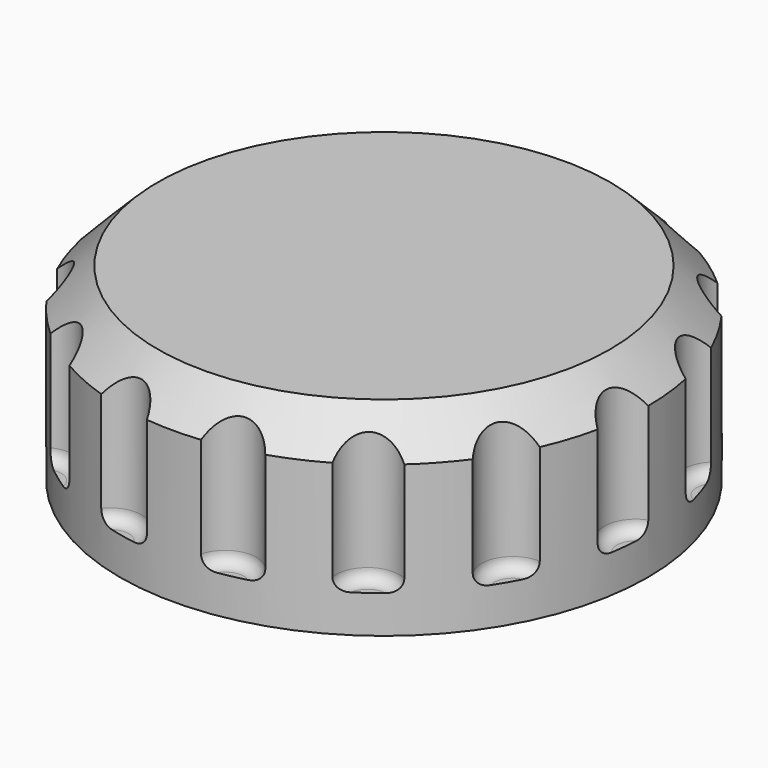
from build123d import *

# Parameters (mm, degrees)
F0_R         = 21
F1_DEPTH     = 15
F2_R         = 2.5
F3_DEPTH     = 12
F4_T3_ANGLE  = 241.487040257
F4_S4_R      = 21
F4_T5_DEPTH  = 5
F4_T8_ANGLE  = 241.487040257
F4_S9_R      = 21
F4_T10_DEPTH = 5
F4_T13_ANGLE = 241.487040257
F4_S14_R     = 21
F4_T15_DEPTH = 5
F4_T18_ANGLE = 241.487040257
F4_S19_R     = 21
F4_T20_DEPTH = 5
F4_T23_ANGLE = 241.487040257
F4_S24_R     = 21
F4_T25_DEPTH = 5
F4_T28_ANGLE = 241.487040257
F4_S29_R     = 21
F4_T30_DEPTH = 5
F4_T33_ANGLE = 241.487040257
F4_S34_R     = 21
F4_T35_DEPTH = 5
F4_T38_ANGLE = 241.487040257
F4_S39_R     = 21
F4_T40_DEPTH = 5
F4_T43_ANGLE = 241.487040257
F4_S44_R     = 21
F4_T45_DEPTH = 5
F4_T48_ANGLE = 241.487040257
F4_S49_R     = 21
F4_T50_DEPTH = 5
F4_T53_ANGLE = 241.487040257
F4_S54_R     = 21
F4_T55_DEPTH = 5
F4_T58_ANGLE = 241.487040257
F4_S59_R     = 21
F4_T60_DEPTH = 5
F4_T63_ANGLE = 241.487040257
F4_S64_R     = 21
F4_T65_DEPTH = 5
F4_T68_ANGLE = 241.487040257
F4_S69_R     = 21
F4_T70_DEPTH = 5
F4_T73_ANGLE = 241.487040257
F4_S74_R     = 21
F4_T75_DEPTH = 5
F5_T2_ANGLE  = 53.8780203583
F5_T4_ANGLE  = 53.8780203583
F5_T6_ANGLE  = 53.8780203583
F5_T8_ANGLE  = 53.8780203583
F5_T10_ANGLE = 53.8780203583
F5_T12_ANGLE = 53.8780203583
F5_T14_ANGLE = 53.8780203583
F5_T16_ANGLE = 53.8780203583
F5_T18_ANGLE = 53.8780203583
F5_T20_ANGLE = 53.8780203583
F5_T22_ANGLE = 53.8780203583
F5_T24_ANGLE = 53.8780203583
F5_T26_ANGLE = 53.8780203583
F5_T28_ANGLE = 53.8780203583
F5_T30_ANGLE = 53.8780203583


# Not quite as in the source:
# - a fillet or chamfer that OpenCascade refuses, or shapes differently, is made with other operations: its cross-section is extruded or revolved along the edge and cut away or added


with BuildPart() as f1:
    # F0 (on Top) → F1 (new body)
    with BuildSketch(Plane.XY):
        Circle(F0_R)
    extrude(amount=F1_DEPTH)

    # F2 (on face) → F3 (cut)
    with BuildSketch(Plane.XY.offset(15)):
        with Locations((0, 22)):
            Circle(F2_R)
        with Locations((-8.9482061477, 20.0980000681)):
            Circle(F2_R)
        with Locations((-16.3491861605, 14.7208733399)):
            Circle(F2_R)
        with Locations((-20.9232433585, 6.7983738762)):
            Circle(F2_R)
        with Locations((-21.8794816981, -2.2996261919)):
            Circle(F2_R)
        with Locations((-19.0525588833, -11)):
            Circle(F2_R)
        with Locations((-12.9312755504, -17.7983738762)):
            Circle(F2_R)
        with Locations((-4.574057198, -21.5192472161)):
            Circle(F2_R)
        with Locations((4.574057198, -21.5192472161)):
            Circle(F2_R)
        with Locations((12.9312755504, -17.7983738762)):
            Circle(F2_R)
        with Locations((19.0525588833, -11)):
            Circle(F2_R)
        with Locations((21.8794816981, -2.2996261919)):
            Circle(F2_R)
        with Locations((20.9232433585, 6.7983738762)):
            Circle(F2_R)
        with Locations((16.3491861605, 14.7208733399)):
            Circle(F2_R)
        with Locations((8.9482061477, 20.0980000681)):
            Circle(F2_R)
    extrude(amount=-F3_DEPTH, mode=Mode.SUBTRACT)

    # F4: fillet of radius 1 on 15 edges, made by hand


with BuildPart() as f4_tool1:
    # F4_s2 → F4_t3 (revolve)
    with BuildSketch(Plane(origin=(15.4399982509, 10.9145304871, 0), x_dir=(0, 0, 1), z_dir=(0.8165762777, 0.5772375445, 0))):
        with BuildLine():
            ThreePointArc((3, -12.7463095395), (3.2928932188, -13.4534163207), (4, -13.7463095395))
            Line((4, -13.7463095395), (3, -13.7463095395))
            Line((3, -13.7463095395), (3, -12.7463095395))
        make_face()
    revolve(axis=Axis((8.9482061477, 20.0980000681, 3), (0, 0, 1)), revolution_arc=F4_T3_ANGLE)

    # F4_s4 → F4_t5 (intersect, symmetric)
    with BuildSketch(Plane.XY.offset(3.9)):
        Circle(F4_S4_R)
    extrude(amount=F4_T5_DEPTH, both=True, mode=Mode.INTERSECT)


with BuildPart() as f4_tool6:
    # F4_s7 → F4_t8 (revolve)
    with BuildSketch(Plane(origin=(18.5444797592, 3.6909066911, 0), x_dir=(0, 0, 1), z_dir=(0.9807632104, 0.1952012428, 0))):
        with BuildLine():
            ThreePointArc((3, -12.7463095395), (3.2928932188, -13.4534163207), (4, -13.7463095395))
            Line((4, -13.7463095395), (3, -13.7463095395))
            Line((3, -13.7463095395), (3, -12.7463095395))
        make_face()
    revolve(axis=Axis((16.3491861605, 14.7208733399, 3), (0, 0, 1)), revolution_arc=F4_T8_ANGLE)

    # F4_s9 → F4_t10 (intersect, symmetric)
    with BuildSketch(Plane.XY.offset(3.9)):
        Circle(F4_S9_R)
    extrude(amount=F4_T10_DEPTH, both=True, mode=Mode.INTERSECT)


with BuildPart() as f4_tool11:
    # F4_s12 → F4_t13 (revolve)
    with BuildSketch(Plane(origin=(18.4424522458, -4.1709084026, 0), x_dir=(0, 0, 1), z_dir=(0.9753672741, -0.2205871272, 0))):
        with BuildLine():
            ThreePointArc((3, -12.7463095395), (3.2928932188, -13.4534163207), (4, -13.7463095395))
            Line((4, -13.7463095395), (3, -13.7463095395))
            Line((3, -13.7463095395), (3, -12.7463095395))
        make_face()
    revolve(axis=Axis((20.9232433585, 6.7983738762, 3), (0, 0, 1)), revolution_arc=F4_T13_ANGLE)

    # F4_s14 → F4_t15 (intersect, symmetric)
    with BuildSketch(Plane.XY.offset(3.9)):
        Circle(F4_S14_R)
    extrude(amount=F4_T15_DEPTH, both=True, mode=Mode.INTERSECT)


with BuildPart() as f4_tool16:
    # F4_s17 → F4_t18 (revolve)
    with BuildSketch(Plane(origin=(15.1515571947, -11.311535542, 0), x_dir=(0, 0, 1), z_dir=(0.8013214751, -0.5982339789, 0))):
        with BuildLine():
            ThreePointArc((4, -13.7463095395), (3.2928932188, -13.4534163207), (3, -12.7463095395))
            Line((3, -12.7463095395), (3, -13.7463095395))
            Line((3, -13.7463095395), (4, -13.7463095395))
        make_face()
    revolve(axis=Axis((21.8794816981, -2.2996261919, 3), (0, 0, 1)), revolution_arc=F4_T18_ANGLE)

    # F4_s19 → F4_t20 (intersect, symmetric)
    with BuildSketch(Plane.XY.offset(3.5)):
        Circle(F4_S19_R)
    extrude(amount=F4_T20_DEPTH, both=True, mode=Mode.INTERSECT)


with BuildPart() as f4_tool21:
    # F4_s22 → F4_t23 (revolve)
    with BuildSketch(Plane(origin=(1.7322615467, -18.8286959632, 0), x_dir=(0, 0, 1), z_dir=(0.0916142387, -0.9957945728, 0))):
        with BuildLine():
            ThreePointArc((3, -12.7463095395), (3.2928932188, -13.4534163207), (4, -13.7463095395))
            Line((4, -13.7463095395), (3, -13.7463095395))
            Line((3, -13.7463095395), (3, -12.7463095395))
        make_face()
    revolve(axis=Axis((12.9312755504, -17.7983738762, 3), (0, 0, 1)), revolution_arc=F4_T23_ANGLE)

    # F4_s24 → F4_t25 (intersect, symmetric)
    with BuildSketch(Plane.XY.offset(3.9)):
        Circle(F4_S24_R)
    extrude(amount=F4_T25_DEPTH, both=True, mode=Mode.INTERSECT)


with BuildPart() as f4_tool26:
    # F4_s27 → F4_t28 (revolve)
    with BuildSketch(Plane(origin=(9.240820257, -16.4962954241, 0), x_dir=(0, 0, 1), z_dir=(0.4887199134, -0.8724407408, 0))):
        with BuildLine():
            ThreePointArc((3, -12.7463095395), (3.2928932188, -13.4534163207), (4, -13.7463095395))
            Line((4, -13.7463095395), (3, -13.7463095395))
            Line((3, -13.7463095395), (3, -12.7463095395))
        make_face()
    revolve(axis=Axis((19.0525588833, -11, 3), (0, 0, 1)), revolution_arc=F4_T28_ANGLE)

    # F4_s29 → F4_t30 (intersect, symmetric)
    with BuildSketch(Plane.XY.offset(3.9)):
        Circle(F4_S29_R)
    extrude(amount=F4_T30_DEPTH, both=True, mode=Mode.INTERSECT)


with BuildPart() as f4_tool31:
    # F4_s32 → F4_t33 (revolve)
    with BuildSketch(Plane(origin=(-6.0758209221, -17.905443917, 0), x_dir=(0, 0, 1), z_dir=(-0.3213323701, -0.9469664767, 0))):
        with BuildLine():
            ThreePointArc((3, -12.7463095395), (3.2928932188, -13.4534163207), (4, -13.7463095395))
            Line((4, -13.7463095395), (3, -13.7463095395))
            Line((3, -13.7463095395), (3, -12.7463095395))
        make_face()
    revolve(axis=Axis((4.574057198, -21.5192472161, 3), (0, 0, 1)), revolution_arc=F4_T33_ANGLE)

    # F4_s34 → F4_t35 (intersect, symmetric)
    with BuildSketch(Plane.XY.offset(3.9)):
        Circle(F4_S34_R)
    extrude(amount=F4_T35_DEPTH, both=True, mode=Mode.INTERSECT)


with BuildPart() as f4_tool36:
    # F4_s37 → F4_t38 (revolve)
    with BuildSketch(Plane(origin=(-12.8333387564, -13.8861779516, 0), x_dir=(0, 0, 1), z_dir=(-0.6787176929, -0.7343992738, 0))):
        with BuildLine():
            ThreePointArc((3, -12.7463095395), (3.2928932188, -13.4534163207), (4, -13.7463095395))
            Line((4, -13.7463095395), (3, -13.7463095395))
            Line((3, -13.7463095395), (3, -12.7463095395))
        make_face()
    revolve(axis=Axis((-4.574057198, -21.5192472161, 3), (0, 0, 1)), revolution_arc=F4_T38_ANGLE)

    # F4_s39 → F4_t40 (intersect, symmetric)
    with BuildSketch(Plane.XY.offset(3.9)):
        Circle(F4_S39_R)
    extrude(amount=F4_T40_DEPTH, both=True, mode=Mode.INTERSECT)


with BuildPart() as f4_tool41:
    # F4_s42 → F4_t43 (revolve)
    with BuildSketch(Plane(origin=(-1.7322615467, -18.8286959632, 0), x_dir=(0, 0, 1), z_dir=(-0.0916142387, -0.9957945728, 0))):
        with BuildLine():
            ThreePointArc((3, 12.7463095395), (3.2928932188, 13.4534163207), (4, 13.7463095395))
            Line((4, 13.7463095395), (3, 13.7463095395))
            Line((3, 13.7463095395), (3, 12.7463095395))
        make_face()
    revolve(axis=Axis((-12.9312755504, -17.7983738762, 3), (0, 0, -1)), revolution_arc=F4_T43_ANGLE)

    # F4_s44 → F4_t45 (intersect, symmetric)
    with BuildSketch(Plane.XY.offset(3.9)):
        Circle(F4_S44_R)
    extrude(amount=F4_T45_DEPTH, both=True, mode=Mode.INTERSECT)


with BuildPart() as f4_tool46:
    # F4_s47 → F4_t48 (revolve)
    with BuildSketch(Plane(origin=(-9.240820257, -16.4962954241, 0), x_dir=(0, 0, 1), z_dir=(-0.4887199134, -0.8724407408, 0))):
        with BuildLine():
            ThreePointArc((3, 12.7463095395), (3.2928932188, 13.4534163207), (4, 13.7463095395))
            Line((4, 13.7463095395), (3, 13.7463095395))
            Line((3, 13.7463095395), (3, 12.7463095395))
        make_face()
    revolve(axis=Axis((-19.0525588833, -11, 3), (0, 0, -1)), revolution_arc=F4_T48_ANGLE)

    # F4_s49 → F4_t50 (intersect, symmetric)
    with BuildSketch(Plane.XY.offset(3.9)):
        Circle(F4_S49_R)
    extrude(amount=F4_T50_DEPTH, both=True, mode=Mode.INTERSECT)


with BuildPart() as f4_tool51:
    # F4_s52 → F4_t53 (revolve)
    with BuildSketch(Plane(origin=(-15.1515571947, -11.311535542, 0), x_dir=(0, 0, 1), z_dir=(-0.8013214751, -0.5982339789, 0))):
        with BuildLine():
            ThreePointArc((3, 12.7463095395), (3.2928932188, 13.4534163207), (4, 13.7463095395))
            Line((4, 13.7463095395), (3, 13.7463095395))
            Line((3, 13.7463095395), (3, 12.7463095395))
        make_face()
    revolve(axis=Axis((-21.8794816981, -2.2996261919, 3), (0, 0, -1)), revolution_arc=F4_T53_ANGLE)

    # F4_s54 → F4_t55 (intersect, symmetric)
    with BuildSketch(Plane.XY.offset(3.9)):
        Circle(F4_S54_R)
    extrude(amount=F4_T55_DEPTH, both=True, mode=Mode.INTERSECT)


with BuildPart() as f4_tool56:
    # F4_s57 → F4_t58 (revolve)
    with BuildSketch(Plane(origin=(-18.4424522458, -4.1709084026, 0), x_dir=(0, 0, 1), z_dir=(-0.9753672741, -0.2205871272, 0))):
        with BuildLine():
            ThreePointArc((3, 12.7463095395), (3.2928932188, 13.4534163207), (4, 13.7463095395))
            Line((4, 13.7463095395), (3, 13.7463095395))
            Line((3, 13.7463095395), (3, 12.7463095395))
        make_face()
    revolve(axis=Axis((-20.9232433585, 6.7983738762, 3), (0, 0, -1)), revolution_arc=F4_T58_ANGLE)

    # F4_s59 → F4_t60 (intersect, symmetric)
    with BuildSketch(Plane.XY.offset(3.9)):
        Circle(F4_S59_R)
    extrude(amount=F4_T60_DEPTH, both=True, mode=Mode.INTERSECT)


with BuildPart() as f4_tool61:
    # F4_s62 → F4_t63 (revolve)
    with BuildSketch(Plane(origin=(-18.5444797592, 3.6909066911, 0), x_dir=(0, 0, 1), z_dir=(-0.9807632104, 0.1952012428, 0))):
        with BuildLine():
            ThreePointArc((3, 12.7463095395), (3.2928932188, 13.4534163207), (4, 13.7463095395))
            Line((4, 13.7463095395), (3, 13.7463095395))
            Line((3, 13.7463095395), (3, 12.7463095395))
        make_face()
    revolve(axis=Axis((-16.3491861605, 14.7208733399, 3), (0, 0, -1)), revolution_arc=F4_T63_ANGLE)

    # F4_s64 → F4_t65 (intersect, symmetric)
    with BuildSketch(Plane.XY.offset(3.9)):
        Circle(F4_S64_R)
    extrude(amount=F4_T65_DEPTH, both=True, mode=Mode.INTERSECT)


with BuildPart() as f4_tool66:
    # F4_s67 → F4_t68 (revolve)
    with BuildSketch(Plane(origin=(2.2202985378, 18.7774012085, 0), x_dir=(0, 0, 1), z_dir=(0.1174250855, 0.9930817435, 0))):
        with BuildLine():
            ThreePointArc((3, -12.7463095395), (3.2928932188, -13.4534163207), (4, -13.7463095395))
            Line((4, -13.7463095395), (3, -13.7463095395))
            Line((3, -13.7463095395), (3, -12.7463095395))
        make_face()
    revolve(axis=Axis((-8.9482061477, 20.0980000681, 3), (0, 0, 1)), revolution_arc=F4_T68_ANGLE)

    # F4_s69 → F4_t70 (intersect, symmetric)
    with BuildSketch(Plane.XY.offset(3.9)):
        Circle(F4_S69_R)
    extrude(amount=F4_T70_DEPTH, both=True, mode=Mode.INTERSECT)


with BuildPart() as f4_tool71:
    # F4_s72 → F4_t73 (revolve)
    with BuildSketch(Plane(origin=(9.6658007771, 16.2509328064, 0), x_dir=(0, 0, 1), z_dir=(0.5111958882, 0.8594642307, 0))):
        with BuildLine():
            ThreePointArc((3, -12.7463095395), (3.2928932188, -13.4534163207), (4, -13.7463095395))
            Line((4, -13.7463095395), (3, -13.7463095395))
            Line((3, -13.7463095395), (3, -12.7463095395))
        make_face()
    revolve(axis=Axis((0, 22, 3), (0, 0, 1)), revolution_arc=F4_T73_ANGLE)

    # F4_s74 → F4_t75 (intersect, symmetric)
    with BuildSketch(Plane.XY.offset(3.9)):
        Circle(F4_S74_R)
    extrude(amount=F4_T75_DEPTH, both=True, mode=Mode.INTERSECT)


with BuildPart() as f1_1:
    add(f1.part)

    # F4_t76: union F4_tool1, F4_tool6, F4_tool11, F4_tool16, F4_tool21, F4_tool26, F4_tool31, F4_tool36, F4_tool41, F4_tool46, F4_tool51, F4_tool56, F4_tool61, F4_tool66, F4_tool71
    add([f4_tool1.part, f4_tool6.part, f4_tool11.part, f4_tool16.part, f4_tool21.part, f4_tool26.part, f4_tool31.part, f4_tool36.part, f4_tool41.part, f4_tool46.part, f4_tool51.part, f4_tool56.part, f4_tool61.part, f4_tool66.part, f4_tool71.part])

    # F5: chamfer of 3 on 15 edges, made by hand

    # F5_s1 → F5_t2 (revolve, cut)
    with BuildSketch(Plane(origin=(0, 0, 0), x_dir=(0, 0, 1), z_dir=(0.4549386949, -0.8905227588, 0))):
        Polygon((12, -21), (15, -18), (15, -21), align=None)
    revolve(axis=Axis((0, 0, 15), (0, 0, 1)), revolution_arc=F5_T2_ANGLE, mode=Mode.SUBTRACT)

    # F5_s3 → F5_t4 (revolve, cut)
    with BuildSketch(Plane(origin=(0, 0, 0), x_dir=(0, 0, 1), z_dir=(-0.3573739754, -0.9339613706, 0))):
        Polygon((12, -21), (15, -18), (15, -21), align=None)
    revolve(axis=Axis((0, 0, 15), (0, 0, 1)), revolution_arc=F5_T4_ANGLE, mode=Mode.SUBTRACT)

    # F5_s5 → F5_t6 (revolve, cut)
    with BuildSketch(Plane(origin=(0, 0, 0), x_dir=(0, 0, 1), z_dir=(0.0533989408, -0.9985732588, 0))):
        Polygon((12, -21), (15, -18), (15, -21), align=None)
    revolve(axis=Axis((0, 0, 15), (0, 0, 1)), revolution_arc=F5_T6_ANGLE, mode=Mode.SUBTRACT)

    # F5_s7 → F5_t8 (revolve, cut)
    with BuildSketch(Plane(origin=(0, 0, 0), x_dir=(0, 0, 1), z_dir=(0.7778154157, -0.6284927836, 0))):
        Polygon((12, -21), (15, -18), (15, -21), align=None)
    revolve(axis=Axis((0, 0, 15), (0, 0, 1)), revolution_arc=F5_T8_ANGLE, mode=Mode.SUBTRACT)

    # F5_s9 → F5_t10 (revolve, cut)
    with BuildSketch(Plane(origin=(0, 0, 0), x_dir=(0, 0, 1), z_dir=(0.9662007849, -0.2577906965, 0))):
        Polygon((12, -21), (15, -18), (15, -21), align=None)
    revolve(axis=Axis((0, 0, 15), (0, 0, 1)), revolution_arc=F5_T10_ANGLE, mode=Mode.SUBTRACT)

    # F5_s11 → F5_t12 (revolve, cut)
    with BuildSketch(Plane(origin=(0, 0, 0), x_dir=(0, 0, 1), z_dir=(0.9875212608, 0.157485744, 0))):
        Polygon((12, -21), (15, -18), (15, -21), align=None)
    revolve(axis=Axis((0, 0, 15), (0, 0, 1)), revolution_arc=F5_T12_ANGLE, mode=Mode.SUBTRACT)

    # F5_s13 → F5_t14 (revolve, cut)
    with BuildSketch(Plane(origin=(0, 0, 0), x_dir=(0, 0, 1), z_dir=(0.8380903393, 0.5455314686, 0))):
        Polygon((12, -21), (15, -18), (15, -21), align=None)
    revolve(axis=Axis((0, 0, 15), (0, 0, 1)), revolution_arc=F5_T14_ANGLE, mode=Mode.SUBTRACT)

    # F5_s15 → F5_t16 (revolve, cut)
    with BuildSketch(Plane(origin=(0, 0, 0), x_dir=(0, 0, 1), z_dir=(0.5437459843, 0.8392498463, 0))):
        Polygon((12, -21), (15, -18), (15, -21), align=None)
    revolve(axis=Axis((0, 0, 15), (0, 0, 1)), revolution_arc=F5_T16_ANGLE, mode=Mode.SUBTRACT)

    # F5_s17 → F5_t18 (revolve, cut)
    with BuildSketch(Plane(origin=(0, 0, 0), x_dir=(0, 0, 1), z_dir=(0.1553830089, 0.9878543013, 0))):
        Polygon((12, -21), (15, -18), (15, -21), align=None)
    revolve(axis=Axis((0, 0, 15), (0, 0, 1)), revolution_arc=F5_T18_ANGLE, mode=Mode.SUBTRACT)

    # F5_s19 → F5_t20 (revolve, cut)
    with BuildSketch(Plane(origin=(0, 0, 0), x_dir=(0, 0, 1), z_dir=(-0.2598471004, 0.9656497732, 0))):
        Polygon((12, -21), (15, -18), (15, -21), align=None)
    revolve(axis=Axis((0, 0, 15), (0, 0, 1)), revolution_arc=F5_T20_ANGLE, mode=Mode.SUBTRACT)

    # F5_s21 → F5_t22 (revolve, cut)
    with BuildSketch(Plane(origin=(0, 0, 0), x_dir=(0, 0, 1), z_dir=(-0.6301472854, 0.7764756266, 0))):
        Polygon((12, -21), (15, -18), (15, -21), align=None)
    revolve(axis=Axis((0, 0, 15), (0, 0, 1)), revolution_arc=F5_T22_ANGLE, mode=Mode.SUBTRACT)

    # F5_s23 → F5_t24 (revolve, cut)
    with BuildSketch(Plane(origin=(0, 0, 0), x_dir=(0, 0, 1), z_dir=(-0.89148928, 0.4530417902, 0))):
        Polygon((12, -21), (15, -18), (15, -21), align=None)
    revolve(axis=Axis((0, 0, 15), (0, 0, 1)), revolution_arc=F5_T24_ANGLE, mode=Mode.SUBTRACT)

    # F5_s25 → F5_t26 (revolve, cut)
    with BuildSketch(Plane(origin=(0, 0, 0), x_dir=(0, 0, 1), z_dir=(-0.9986846792, 0.0512729124, 0))):
        Polygon((12, -21), (15, -18), (15, -21), align=None)
    revolve(axis=Axis((0, 0, 15), (0, 0, 1)), revolution_arc=F5_T26_ANGLE, mode=Mode.SUBTRACT)

    # F5_s27 → F5_t28 (revolve, cut)
    with BuildSketch(Plane(origin=(0, 0, 0), x_dir=(0, 0, 1), z_dir=(-0.9331984246, -0.3593615177, 0))):
        Polygon((12, -21), (15, -18), (15, -21), align=None)
    revolve(axis=Axis((0, 0, 15), (0, 0, 1)), revolution_arc=F5_T28_ANGLE, mode=Mode.SUBTRACT)

    # F5_s29 → F5_t30 (revolve, cut)
    with BuildSketch(Plane(origin=(0, 0, 0), x_dir=(0, 0, 1), z_dir=(-0.7063536845, -0.7078590766, 0))):
        Polygon((12, -21), (15, -18), (15, -21), align=None)
    revolve(axis=Axis((0, 0, 15), (0, 0, 1)), revolution_arc=F5_T30_ANGLE, mode=Mode.SUBTRACT)


solid = f1_1.part
